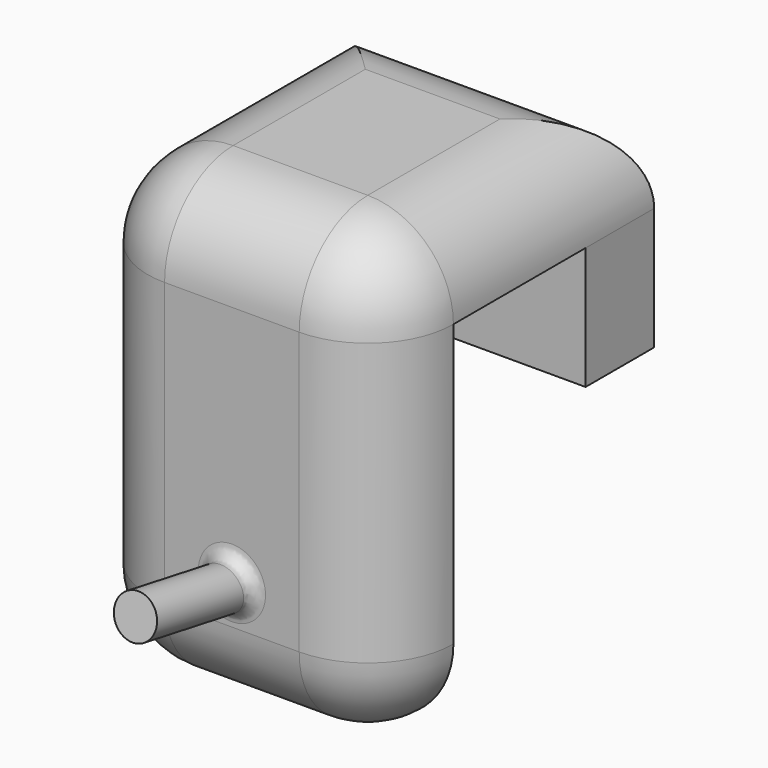
from build123d import *

# Parameters (mm, degrees)
F1_DEPTH      = 25
F5_R          = 6.99999
F6_R          = 1.75
F7_DEPTH      = 10
F7_DEPTH_BACK = 5
F8_R          = 1


# Not quite as in the source:
# - a fillet or chamfer is up to 0.001 mm smaller than in the source, because OpenCascade refuses the exact size


with BuildPart() as f1:
    # F0 (on Right) → F1 (new body)
    with BuildSketch(Plane.YZ):
        Polygon((0, 21.183779), (0, -15.816221), (7, -15.816221), (7, 14.183779), (20.5, 14.183779), (20.5, 4.183779), (27.5, 4.183779), (27.5, 21.183779), align=None)
    extrude(amount=F1_DEPTH)

    # F5 (radius 7 in the source; OpenCascade refuses exactly that, so slightly less here)
    f5_edges = [f1.edges().sort_by_distance(p)[0] for p in [
        (25, 0, 2.683779),
        (12.5, 0, 21.183779),
        (0, 0, 2.683779),
        (12.5, 0, -15.816221),
        (25, 13.75, 21.183779),
        (0, 13.75, 21.183779),
        (25, 3.5, -15.816221),
        (0, 3.5, -15.816221),
        (12.5, 27.5, 21.183779),
    ]]
    fillet(f5_edges, radius=F5_R)

    # F6 (on face) → F7 (join, two sides)
    with BuildSketch(Plane(origin=(0, 0.994632, -0.175381), x_dir=(1, 0, 0), z_dir=(0, -0.984808, 0.173648))) as f7_sk:
        with Locations((12.5, -5.727859)):
            Circle(F6_R)
    extrude(amount=F7_DEPTH)
    extrude(f7_sk.sketch, amount=-F7_DEPTH_BACK)

    # F8
    f8_edges = [f1.edges().sort_by_distance(p)[0] for p in [
        (12.5, 0, -4.039224),
        (12.5, 0, -7.593217),
    ]]
    fillet(f8_edges, radius=F8_R)


solid = f1.part
